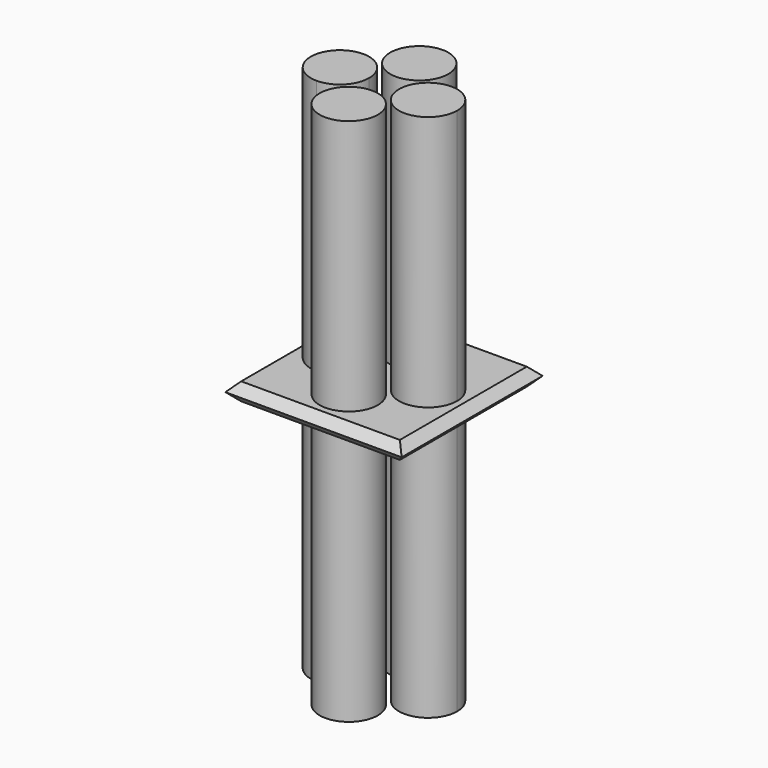
from build123d import *

# Parameters (mm, degrees)
F1_DEPTH = 150
F0_R     = 16.5
F0_W     = 100
F0_H     = 100
F2_DEPTH = 5
F3_SIZE  = 5
F4_SIZE  = 4.99999


# Not quite as in the source:
# - a fillet or chamfer is up to 0.001 mm smaller than in the source, because OpenCascade refuses the exact size


with BuildPart() as f1:
    # F0 (on Top) → F1 (new body, symmetric)
    with BuildSketch(Plane.XY):
        with BuildLine():
            ThreePointArc((-16.5, 25), (0, 8.5), (16.5, 25))
            ThreePointArc((16.5, 25), (0, 41.5), (-16.5, 25))
        make_face()
    extrude(amount=F1_DEPTH, both=True)


with BuildPart() as f1b:
    # F0 (on Top) → F1, piece 2 (new body, symmetric)
    with BuildSketch(Plane.XY):
        with BuildLine():
            ThreePointArc((-25, -16.5), (-13.3327381104, -11.6672618896), (-8.5, 0))
            ThreePointArc((-8.5, 0), (-36.6672618896, 11.6672618896), (-25, -16.5))
        make_face()
    extrude(amount=F1_DEPTH, both=True)


with BuildPart() as f1c:
    # F0 (on Top) → F1, piece 3 (new body, symmetric)
    with BuildSketch(Plane.XY):
        with BuildLine():
            ThreePointArc((25, 16.5), (13.3327381104, -11.6672618896), (41.5, 0))
            ThreePointArc((41.5, 0), (36.6672618896, 11.6672618896), (25, 16.5))
        make_face()
    extrude(amount=F1_DEPTH, both=True)


with BuildPart() as f1d:
    # F0 (on Top) → F1, piece 4 (new body, symmetric)
    with BuildSketch(Plane.XY):
        with Locations((0, -25)):
            Circle(F0_R)
    extrude(amount=F1_DEPTH, both=True)


with BuildPart() as f2:
    # F0 (on Top) → F2 (new body, symmetric)
    with BuildSketch(Plane.XY):
        Rectangle(F0_W, F0_H)
        with Locations((0, -25)):
            Circle(F0_R, mode=Mode.SUBTRACT)
        with BuildLine():
            ThreePointArc((-25, -16.5), (-36.6672618896, 11.6672618896), (-8.5, 0))
            ThreePointArc((-8.5, 0), (-13.3327381104, -11.6672618896), (-25, -16.5))
        make_face(mode=Mode.SUBTRACT)
        with BuildLine():
            ThreePointArc((25, 16.5), (36.6672618896, 11.6672618896), (41.5, 0))
            ThreePointArc((41.5, 0), (13.3327381104, -11.6672618896), (25, 16.5))
        make_face(mode=Mode.SUBTRACT)
        with BuildLine():
            ThreePointArc((-16.5, 25), (0, 41.5), (16.5, 25))
            ThreePointArc((16.5, 25), (0, 8.5), (-16.5, 25))
        make_face(mode=Mode.SUBTRACT)
    extrude(amount=F2_DEPTH, both=True)

    # F3
    f3_edges = [f2.edges().sort_by_distance(p)[0] for p in [
        (0, -50, 5),
        (50, 0, 5),
        (-50, 0, 5),
        (0, 50, 5),
    ]]
    chamfer(f3_edges, length=F3_SIZE)

    # F4 (size 5 in the source; OpenCascade refuses exactly that, so slightly less here)
    f4_edges = [f2.edges().sort_by_distance(p)[0] for p in [
        (0, 50, -5),
        (50, 0, -5),
        (0, -50, -5),
        (-50, 0, -5),
    ]]
    chamfer(f4_edges, length=F4_SIZE)


solid = Compound([f1.part, f1b.part, f1c.part, f1d.part, f2.part])
